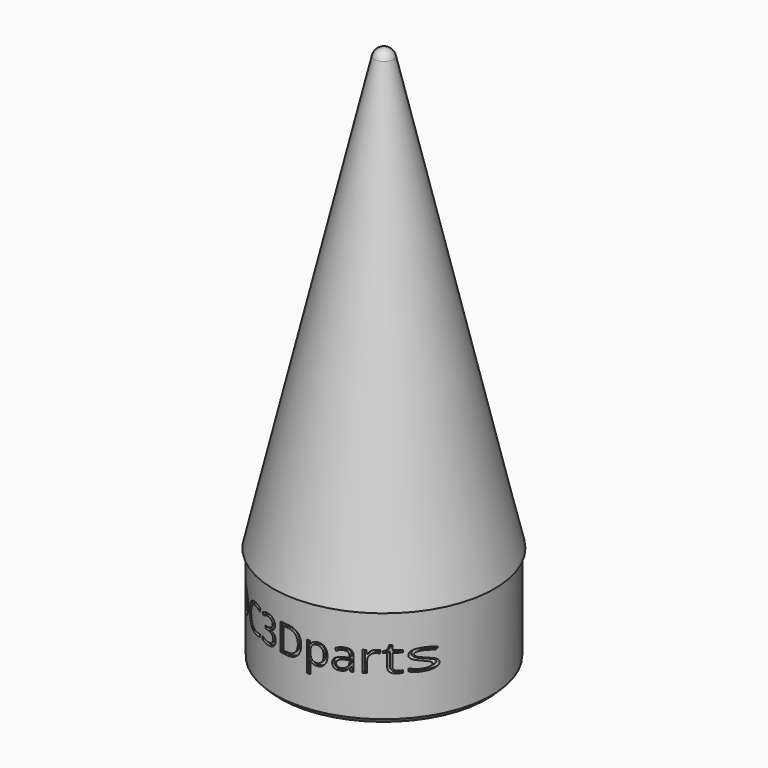
from build123d import *

# Parameters (mm, degrees)
F2_SIZE      = 1.5
F3_SCALE     = 0.848
F5_W         = 27
F5_H         = 36.2020888026
F7_TEXT_SIZE = 9.7222222222
F8_DEPTH     = 35


# Not quite as in the source:
# - Text() gives the source's letters only with a copy of the font that has no kerning and outlines rounded to 1/6400 em; it was checked with that copy


with BuildPart() as f1:
    # F0 (on Front) → F1 (revolve)
    with BuildSketch(Plane.XZ):
        with BuildLine():
            Line((-2.8584917819, 61.9171100258), (-33.35, -68.7499268014))
            Line((-33.35, -68.7499268014), (-32.6, -68.7499268014))
            Line((-32.6, -68.7499268014), (-32.6, -98.7499268014))
            Line((-32.6, -98.7499268014), (0, -98.7499268014))
            Line((0, -98.7499268014), (0, -68.7499268014))
            Line((0, -68.7499268014), (0, 64.1853608159))
            ThreePointArc((0, 64.1853608159), (-1.8245504182, 63.5494055295), (-2.8584917819, 61.9171100258))
        make_face()
    revolve(axis=Axis((0, 0, 9.1068005099), (0, 0, 1)))

    # F2
    f2_edges = [f1.edges().sort_by_distance(p)[0] for p in [
        (32.6, 0, -98.749927),
    ]]
    chamfer(f2_edges, length=F2_SIZE)


with BuildPart() as f1_1:
    # F3: moved
    add(f1.part.scale(F3_SCALE))


with BuildPart() as f6:
    # F5 (on Front) → F6 (revolve)
    with BuildSketch(Plane.XZ):
        with Locations((-13.5, -79.3815848689)):
            Rectangle(F5_W, F5_H)
    revolve(axis=Axis((0, 0, -79.3815848689), (0, 0, -1)))


with BuildPart() as f8:
    # F7 (on offset) → F8 (new body, through all)
    with BuildSketch(Plane.XZ.offset(35)):
        with Locations((-24.3215298089, -72.1694954322)):
            Text('DC3Dparts', F7_TEXT_SIZE, font='Open Sans', text_align=(TextAlign.LEFT, TextAlign.BOTTOM))
    extrude(amount=-F8_DEPTH)

    # F9: cut F6
    add(f6.part, mode=Mode.SUBTRACT)


with BuildPart() as f1_2:
    add(f1_1.part)

    # F10: cut F8
    add(f8.part, mode=Mode.SUBTRACT)


solid = f1_2.part
